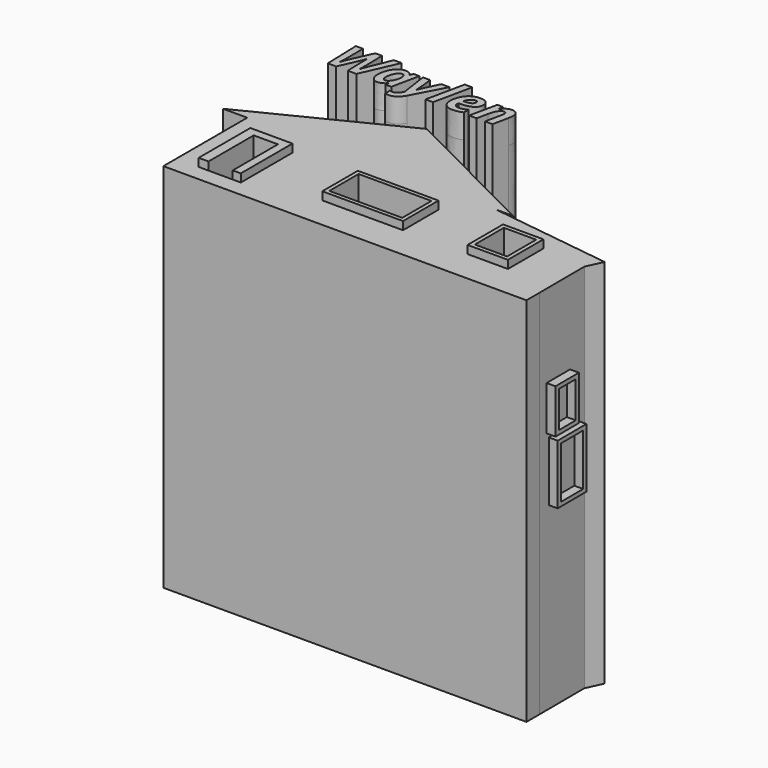
from build123d import *

# Parameters (mm, degrees)
F1_DEPTH      = 914.4
F2_DEPTH      = 12192
F0_W          = 3048
F0_H          = 1676.4
F0_W_2        = 1524
F0_W_3        = 4572
F0_H_2        = 609.6
F0_TEXT_SIZE  = 1928.037405014
F3_DEPTH      = 914.4
F3_DEPTH_BACK = 13106.4
F0_W_4        = 2753.2
F0_H_3        = 1381.6
F0_W_5        = 1219.2
F0_H_4        = 1371.6
F4_DEPTH      = 1219.2
F5_DEPTH      = 914.4
F7_W          = 1110.2677415848
F7_H          = 1675.6055355072
F7_W_2        = 805.4677415848
F7_H_2        = 1370.8055355072
F7_W_3        = 1363.9131616592
F7_H_3        = 2252.0575523376
F7_W_4        = 1059.1131616592
F7_H_4        = 1947.2575523376
F8_DEPTH      = 30.48
F9_W          = 1363.9131616592
F9_H          = 2252.0575523376
F9_W_2        = 1059.1131616592
F9_H_2        = 1947.2575523376
F8_FACE_W     = 1110.2677415848
F8_FACE_H     = 1675.6055355072
F8_FACE_W_2   = 805.4677415848
F8_FACE_H_2   = 1370.8055355072
F10_DEPTH     = 304.8


# Not quite as in the source:
# - a feature of the source that left no trace in its solid (it failed there, or was rolled back) is left out
# - Text() gives the source's letters only with a copy of the font that has no kerning and outlines rounded to 1/6400 em; it was checked with that copy


with BuildPart() as f1:
    # F0 (on Top) → F1 (new body)
    with BuildSketch(Plane.XY):
        Polygon((0, 2286), (4572, 0), (4844.6214078168, 0), (5486.4, 0), (0, 2743.2), align=None)
        Polygon((-5486.4, 0), (-4572, 0), (0, 2286), (0, 2743.2), align=None)
    extrude(amount=F1_DEPTH)

    # F0 (on Top) → F3 (join, two sides)
    with BuildSketch(Plane.XY) as f3_sk:
        Polygon((4572, 0), (0, 0), (-4572, 0), (-4572, -3352.8), (-3724.7197628021, -3352.8), (-3724.7197628021, -914.4), (-2133.6, -914.4), (-2133.6, -3352.8), (4572, -3352.8), (4572, -1090.4856312671), (4572, -545.2428156335), align=None)
        with Locations((1981.2, -1905)):
            Rectangle(F0_W, F0_H, mode=Mode.SUBTRACT)
        Polygon((-4572, 0), (0, 0), (0, 2286), align=None)
        Polygon((0, 2286), (4572, 0), (4844.6214078168, 0), (5486.4, 0), (0, 2743.2), align=None)
        Polygon((4844.6214078168, 0), (4572, 0), (4572, -545.2428156335), align=None)
        Polygon((-5486.4, 0), (-4572, 0), (0, 2286), (0, 2743.2), align=None)
        Polygon((9415.7770338457, -609.6), (4844.6214078168, 0), (4572, -545.2428156335), (9134.1110936733, -1219.2), align=None)
        Polygon((9134.1110936733, -1219.2), (4572, -545.2428156335), (4572, -1090.4856312671), (4572, -3352.8), (9144, -3352.8), align=None)
        with Locations((6705.6, -1905)):
            Rectangle(F0_W_2, F0_H, mode=Mode.SUBTRACT)
        Polygon((-3724.7197628021, -3352.8), (-4572, -3352.8), (-4572, -3962.4), (4572, -3962.4), (4572, -3352.8), (-2133.6, -3352.8), (-2438.4, -3352.8), (-3352.8, -3352.8), align=None)
        with Locations((6858, -3657.6)):
            Rectangle(F0_W_3, F0_H_2)
        with Locations((-5102.4432182312, 4196.310043335)):
            Text('Waylen', F0_TEXT_SIZE, font='Open Sans', font_style=FontStyle.BOLDITALIC, text_align=(TextAlign.LEFT, TextAlign.BOTTOM))
    extrude(amount=F3_DEPTH)
    extrude(f3_sk.sketch, amount=-F3_DEPTH_BACK)

    # F0 (on Top) → F4 (join)
    with BuildSketch(Plane.XY):
        with Locations((1981.2, -1905)):
            Rectangle(F0_W, F0_H)
        with Locations((1981.2, -1905)):
            Rectangle(F0_W_4, F0_H_3, mode=Mode.SUBTRACT)
        with Locations((6705.6, -1905)):
            Rectangle(F0_W_2, F0_H)
        with Locations((6705.6, -1905)):
            Rectangle(F0_W_5, F0_H_4, mode=Mode.SUBTRACT)
        Polygon((-3724.7197628021, -914.4), (-3724.7197628021, -3352.8), (-3352.8, -3352.8), (-3352.8, -1219.2), (-2438.4, -1219.2), (-2438.4, -3352.8), (-2133.6, -3352.8), (-2133.6, -914.4), align=None)
    extrude(amount=F4_DEPTH)

    # F0 (on Top) → F5 (join)
    with BuildSketch(Plane.XY):
        Polygon((0, 2286), (0, 0), (4572, 0), align=None)
        Polygon((-4572, 0), (0, 0), (0, 2286), align=None)
    extrude(amount=F5_DEPTH)

    # F7 (on face) → F8 (join)
    with BuildSketch(Plane(origin=(9128.2641985791, 42.3080941063, 0), x_dir=(-0.0046347957, 0.9999892593, 0), z_dir=(0.9999892593, 0.0046347957, 0))):
        with Locations((-2494.7018111229, -3063.377737999)):
            Rectangle(F7_W, F7_H)
        with Locations((-2494.7018111229, -3063.377737999)):
            Rectangle(F7_W_2, F7_H_2, mode=Mode.SUBTRACT)
        with Locations((-2266.0266840935, -5201.79438591)):
            Rectangle(F7_W_3, F7_H_3)
        with Locations((-2266.0266840935, -5201.79438591)):
            Rectangle(F7_W_4, F7_H_4, mode=Mode.SUBTRACT)
    extrude(amount=F8_DEPTH)

    # F9 (on face) + F8_face (on face) → F10 (join)
    with BuildSketch(Plane(origin=(9158.7438712018, 42.4493626794, 0), x_dir=(-0.0046347957, 0.9999892593, 0), z_dir=(0.9999892593, 0.0046347957, 0))):
        with Locations((-2266.0266840935, -5201.79438591)):
            Rectangle(F9_W, F9_H)
        with Locations((-2266.0266840935, -5201.79438591)):
            Rectangle(F9_W_2, F9_H_2, mode=Mode.SUBTRACT)
    with BuildSketch(Plane(origin=(9169.246441941, -2223.5529826485, -5201.79438591), x_dir=(-0.0046347957, 0.9999892593, 0), z_dir=(0.9999892593, 0.0046347957, 0))):
        with Locations((-228.6751270294, 2138.4166479111)):
            Rectangle(F8_FACE_W, F8_FACE_H)
        with Locations((-228.6751270294, 2138.4166479111)):
            Rectangle(F8_FACE_W_2, F8_FACE_H_2, mode=Mode.SUBTRACT)
    extrude(amount=F10_DEPTH)


with BuildPart() as f2:
    # F0 (on Top) → F2 (new body)
    with BuildSketch(Plane.XY):
        Polygon((-4572, 0), (0, 0), (0, 2286), align=None)
        Polygon((0, 2286), (0, 0), (4572, 0), align=None)
    extrude(amount=-F2_DEPTH)


solid = Compound([f1.part, f2.part])
